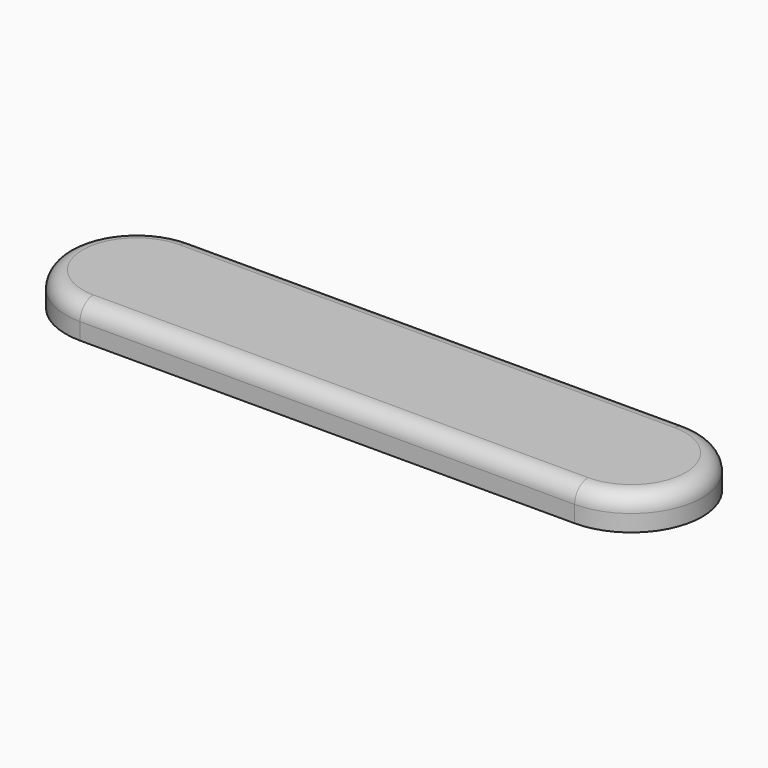
from build123d import *

# Parameters (mm, degrees)
F0_W     = 44.358856976
F0_H     = 12.7014997415
F1_DEPTH = 1.5
F2_R     = 1.5


# Not quite as in the source:
# - a feature names something its author has since deleted; it is built from what else it names


with BuildPart() as f1:
    # F0 (on Top) → F1 (new body, symmetric)
    with BuildSketch(Plane.XY):
        with Locations((10.1427063346, 0.782278832)):
            Rectangle(F0_W, F0_H)
        with BuildLine():
            ThreePointArc((-12.0367221534, 7.1330287028), (-18.3874720242, 0.782278832), (-12.0367221534, -5.5684710387))
            Line((-12.0367221534, -5.5684710387), (-12.0367221534, 7.1330287028))
        make_face()
        with BuildLine():
            Line((32.3221348226, 7.1330287028), (32.3221348226, -5.5684710387))
            ThreePointArc((32.3221348226, -5.5684710387), (38.6728846934, 0.782278832), (32.3221348226, 7.1330287028))
        make_face()
    extrude(amount=F1_DEPTH, both=True)

    # F2
    f2_edges = [f1.edges().sort_by_distance(p)[0] for p in [
        (10.142706, -5.568471, 1.5),
        (10.142706, 7.133029, 1.5),
        (38.672885, 0.782279, 1.5),
    ]]
    fillet(f2_edges, radius=F2_R)


solid = f1.part
